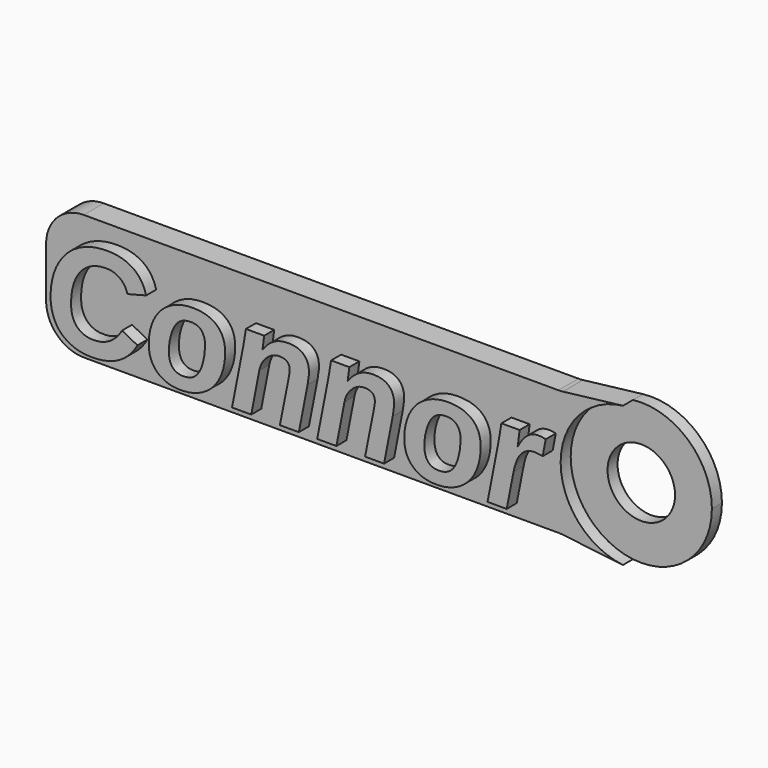
from build123d import *

# Parameters (mm, degrees)
F0_TEXT_SIZE = 11.1111111111
F1_DEPTH     = 1
F2_R         = 2.69
F3_DEPTH     = 2
F4_R         = 3
F5_R         = 5.625
F6_DEPTH     = 1


# Not quite as in the source:
# - Text() gives the source's letters only with a copy of the font that has no kerning and outlines rounded to 1/6400 em; it was checked with that copy


with BuildPart() as f1:
    # F0 (on Front) → F1 (new body)
    with BuildSketch(Plane.XZ):
        with Locations((-20.3845486111, -8)):
            Text('Connor', F0_TEXT_SIZE, font='Arimo', font_style=FontStyle.BOLDITALIC, text_align=(TextAlign.LEFT, TextAlign.BOTTOM))
    extrude(amount=F1_DEPTH)


with BuildPart() as f3:
    # F2 (on Front) → F3 (new body)
    with BuildSketch(Plane.XZ):
        with BuildLine():
            Line((-21, -9), (20, -9))
            Line((20, -9), (24.9655172414, -9.5862068966))
            ThreePointArc((24.9655172414, -9.5862068966), (20, -4), (24.9655172414, 1.5862068966))
            Line((24.9655172414, 1.5862068966), (20, 1))
            Line((20, 1), (-21, 1))
            Line((-21, 1), (-21, -9))
        make_face()
        with BuildLine():
            ThreePointArc((24.9655172414, 1.5862068966), (20, -4), (24.9655172414, -9.5862068966))
            ThreePointArc((24.9655172414, -9.5862068966), (29.3620465934, -8.2041774176), (31.25, -4))
            ThreePointArc((31.25, -4), (29.3620465934, 0.2041774176), (24.9655172414, 1.5862068966))
        make_face()
        with Locations((25.625, -4)):
            Circle(F2_R, mode=Mode.SUBTRACT)
    extrude(amount=-F3_DEPTH)

    # F4
    f4_edges = [f3.edges().sort_by_distance(p)[0] for p in [
        (-21, 1, 1),
        (-21, 1, -9),
        (20, 1, -9),
        (20, 1, 1),
    ]]
    fillet(f4_edges, radius=F4_R)

    # F5 (on face) → F6 (cut)
    with BuildSketch(Plane.XZ):
        with Locations((25.625, -4)):
            Circle(F5_R)
    extrude(amount=-F6_DEPTH, mode=Mode.SUBTRACT)


solid = Compound([f1.part, f3.part])
